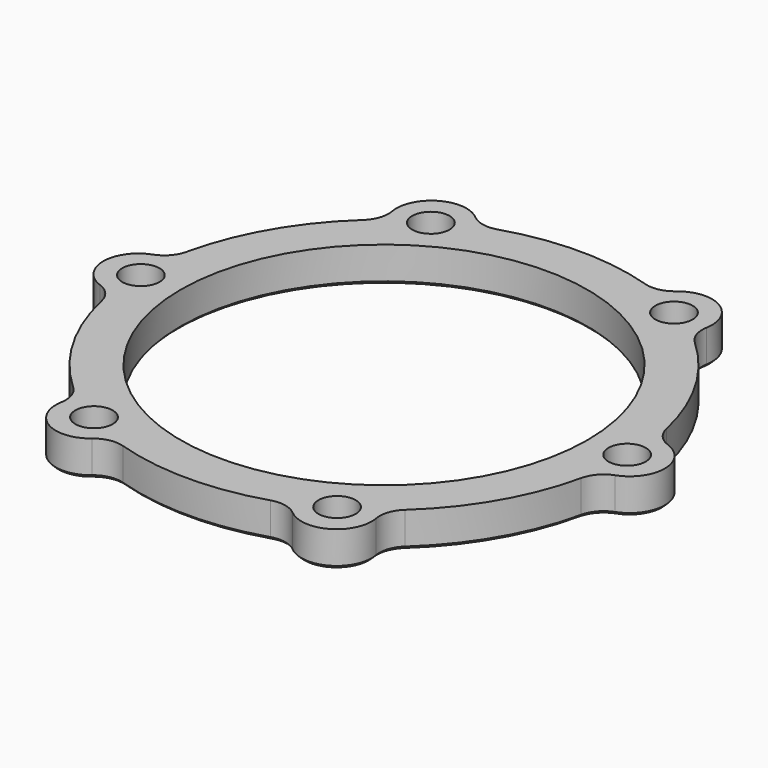
from build123d import *

# Parameters (mm, degrees)
F0_R            = 44.45
F0_R_2          = 36.83
F1_DEPTH        = 6.35
F2_R            = 6.35
F3_DEPTH        = 6.35
F3_COPIES_COUNT = 6
F5_D            = 6.7564
F5_DEPTH        = 12.7
F5_TIP          = 2.0298273432
F5_COPIES_COUNT = 6
F7_R            = 5.08
F8_SIZE         = 0.508


# Not quite as in the source:
# - a pattern or mirror of a feature is missing from the dataset's text; its kind, count and spacing are read off the source's solid


with BuildPart() as f1:
    # F0 (on Top) → F1 (new body)
    with BuildSketch(Plane.XY):
        Circle(F0_R)
        Circle(F0_R_2, mode=Mode.SUBTRACT)
    extrude(amount=F1_DEPTH)

    # F2 (on face) → F3 (join)
    with BuildSketch(Plane.XY.offset(6.35)):
        with Locations((44.45, 0)):
            Circle(F2_R)
    f3 = extrude(amount=-F3_DEPTH)

    # F3_copies: F3 ×6 about axis
    f3_copies_axis = Axis((0, 0, 0), (0, 0, 1))
    for i in range(1, F3_COPIES_COUNT):
        add(f3.rotate(f3_copies_axis, i * 360 / F3_COPIES_COUNT))

    # F5
    with Locations(Plane(origin=(0, 0, 0), x_dir=(1, 0, 0), z_dir=(0, 0, -1))):
        with Locations((43.9964285714, 0)):
            f5 = Hole(F5_D / 2, depth=F5_DEPTH)
            with Locations((0, 0, -(F5_DEPTH + F5_TIP / 2))):  # 118° drill point
                Cone(0, F5_D / 2, F5_TIP, mode=Mode.SUBTRACT)

    # F5_copies: F5 ×6 about axis
    f5_copies_axis = Axis((0, 0, 0), (0, 0, 1))
    for i in range(1, F5_COPIES_COUNT):
        add(f5.rotate(f5_copies_axis, i * 360 / F5_COPIES_COUNT), mode=Mode.SUBTRACT)

    # F7
    f7_edges = [f1.edges().sort_by_distance(p)[0] for p in [
        (43.996429, -6.33378, 3.175),
        (43.996429, 6.33378, 3.175),
        (27.483429, 34.935135, 3.175),
        (27.483429, -34.935135, 3.175),
        (16.513, 41.268915, 3.175),
        (16.513, -41.268915, 3.175),
        (-16.513, 41.268915, 3.175),
        (-16.513, -41.268915, 3.175),
        (-27.483429, 34.935135, 3.175),
        (-27.483429, -34.935135, 3.175),
        (-43.996429, 6.33378, 3.175),
        (-43.996429, -6.33378, 3.175),
    ]]
    fillet(f7_edges, radius=F7_R)

    # F8
    f8_edges = [f1.edges().sort_by_distance(p)[0] for p in [
        (50.8, 0, 0),
        (44.533522, 7.391873, 0),
        (44.533522, -7.391873, 0),
        (38.494829, 22.225, 0),
        (38.494829, -22.225, 0),
        (28.668311, 34.871224, 0),
        (28.668311, -34.871224, 0),
        (25.4, 43.994091, 0),
        (25.4, -43.994091, 0),
        (15.865211, 42.263098, 0),
        (15.865211, -42.263098, 0),
        (0, 44.45, 0),
        (0, -44.45, 0),
        (-15.865211, 42.263098, 0),
        (-15.865211, -42.263098, 0),
        (-25.4, 43.994091, 0),
        (-25.4, -43.994091, 0),
        (-28.668311, 34.871224, 0),
        (-28.668311, -34.871224, 0),
        (-38.494829, 22.225, 0),
        (-38.494829, -22.225, 0),
        (-44.533522, 7.391873, 0),
        (-44.533522, -7.391873, 0),
        (-50.8, 0, 0),
        (-20.309114, -35.176418, 0),
        (20.309114, -35.176418, 0),
        (-40.618229, 0, 0),
        (-36.83, 0, 0),
        (-20.309114, 35.176418, 0),
        (40.618229, 0, 0),
        (20.309114, 35.176418, 0),
    ]]
    chamfer(f8_edges, length=F8_SIZE)


solid = f1.part
